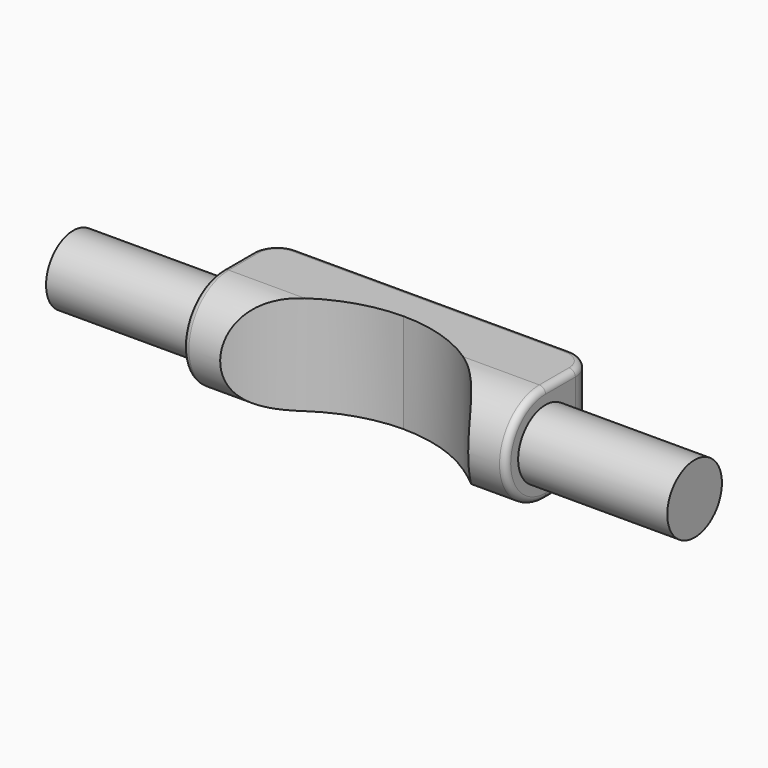
from build123d import *

# Parameters (mm, degrees)
F0_R          = 2.75
F1_DEPTH      = 25
F2_DEPTH      = 13
F3_R          = 2
F5_DEPTH      = 25
F5_DEPTH_BACK = 25
F7_R          = 0.5


with BuildPart() as f1:
    # F0 (on Right) → F1 (new body)
    with BuildSketch(Plane.YZ):
        Circle(F0_R)
    extrude(amount=F1_DEPTH)

    # F0 (on Right) → F2 (join)
    with BuildSketch(Plane.YZ):
        with BuildLine():
            ThreePointArc((0, -4), (2.8284271247, -2.8284271247), (4, 0))
            ThreePointArc((4, 0), (2.8284271247, 2.8284271247), (0, 4))
            ThreePointArc((0, 4), (-4, 0), (0, -4))
        make_face()
        Circle(F0_R, mode=Mode.SUBTRACT)
        with BuildLine():
            ThreePointArc((0, 4), (2.8284271247, 2.8284271247), (4, 0))
            ThreePointArc((4, 0), (2.8284271247, -2.8284271247), (0, -4))
            Line((0, -4), (5, -4))
            Line((5, -4), (5, 4))
            Line((5, 4), (0, 4))
        make_face()
    extrude(amount=F2_DEPTH)

    # F3
    f3_edges = [f1.edges().sort_by_distance(p)[0] for p in [
        (13, 5, 0),
    ]]
    fillet(f3_edges, radius=F3_R)

    # F4 (on Top) → F5 (cut, two sides)
    with BuildSketch(Plane.XY) as f5_sk:
        with BuildLine():
            Line((0, 1.9661990377), (0, -4.0338009623))
            Line((0, -4.0338009623), (10, -4.0338009623))
            ThreePointArc((10, -4.0338009623), (5.8309518948, 0.3511188625), (0, 1.9661990377))
        make_face()
    extrude(amount=F5_DEPTH, mode=Mode.SUBTRACT)
    extrude(f5_sk.sketch, amount=-F5_DEPTH_BACK, mode=Mode.SUBTRACT)

    # F6: F1 across face


with BuildPart() as f1_1:
    add(f1.part)
    add(f1.part.mirror(Plane(origin=(0, 3.4830995189, 0), x_dir=(0, -1, 0), z_dir=(-1, 0, 0))))

    # F7
    f7_edges = [f1_1.edges().sort_by_distance(p)[0] for p in [
        (13, -4, 0),
        (-13, -4, 0),
        (13, 1.5, -4),
        (13, 1.5, 4),
        (0, 5, 4),
        (12.414214, 4.414214, 4),
        (-13, 1.5, 4),
        (-12.414214, 4.414214, 4),
        (-12.414214, 4.414214, -4),
        (-13, 1.5, -4),
        (0, 5, -4),
        (12.414214, 4.414214, -4),
    ]]
    fillet(f7_edges, radius=F7_R)


solid = f1_1.part
